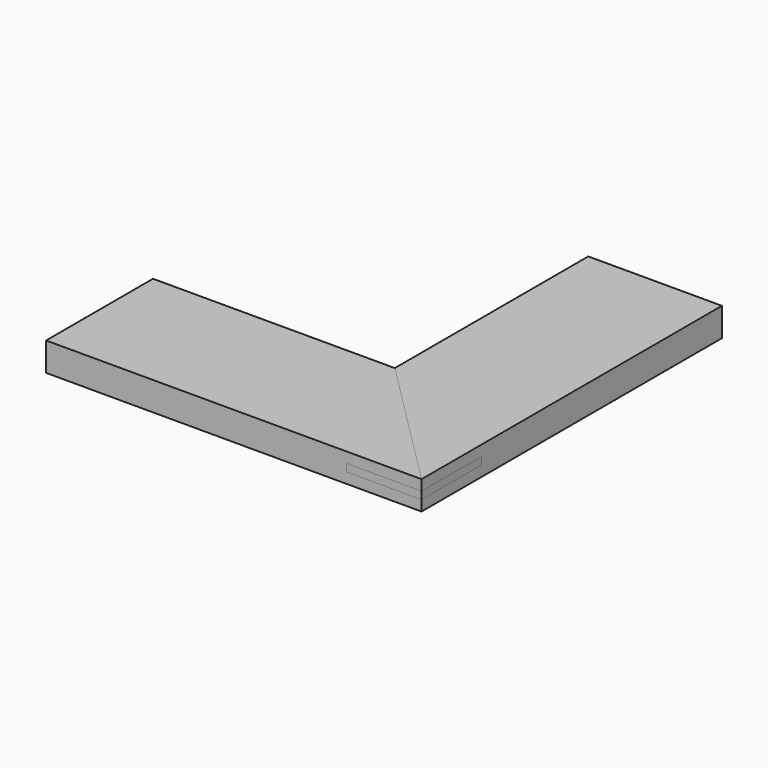
from build123d import *

# Parameters (mm, degrees)
F0_W     = 250
F0_H     = 89
F1_DEPTH = 19
F2_W     = 89
F2_H     = 250
F3_DEPTH = 19
F5_DEPTH = 19.001
F9_DEPTH = 2.5


with BuildPart() as f1:
    # F0 (on Top) → F1 (new body)
    with BuildSketch(Plane.XY):
        with Locations((-125, 44.5)):
            Rectangle(F0_W, F0_H)
    extrude(amount=F1_DEPTH)

    # F4 (on face) → F5 (cut, through all)
    with BuildSketch(Plane.XY.offset(19)):
        Polygon((-89, 89), (0, 0), (0, 89), align=None)
    extrude(amount=-F5_DEPTH, mode=Mode.SUBTRACT)


with BuildPart() as f3:
    # F2 (on Top) → F3 (new body)
    with BuildSketch(Plane.XY):
        with Locations((-44.5, 125)):
            Rectangle(F2_W, F2_H)
    extrude(amount=F3_DEPTH)

    # F6: cut F1
    add(f1.part, mode=Mode.SUBTRACT)


with BuildPart() as f9:
    # F8 (on mid) → F9 (new body, symmetric)
    with BuildSketch(Plane(origin=(0, 0, 9.5), x_dir=(1, 0, 0), z_dir=(0, 0, -1))):
        Polygon((-50, 0), (0, -50), (0, 0), align=None)
    extrude(amount=F9_DEPTH, both=True)


with BuildPart() as f1_1:
    add(f1.part)

    # F10: cut F9
    add(f9.part, mode=Mode.SUBTRACT)


with BuildPart() as f3_1:
    add(f3.part)

    # F10: cut F9
    add(f9.part, mode=Mode.SUBTRACT)


solid = Compound([f9.part, f1_1.part, f3_1.part])
